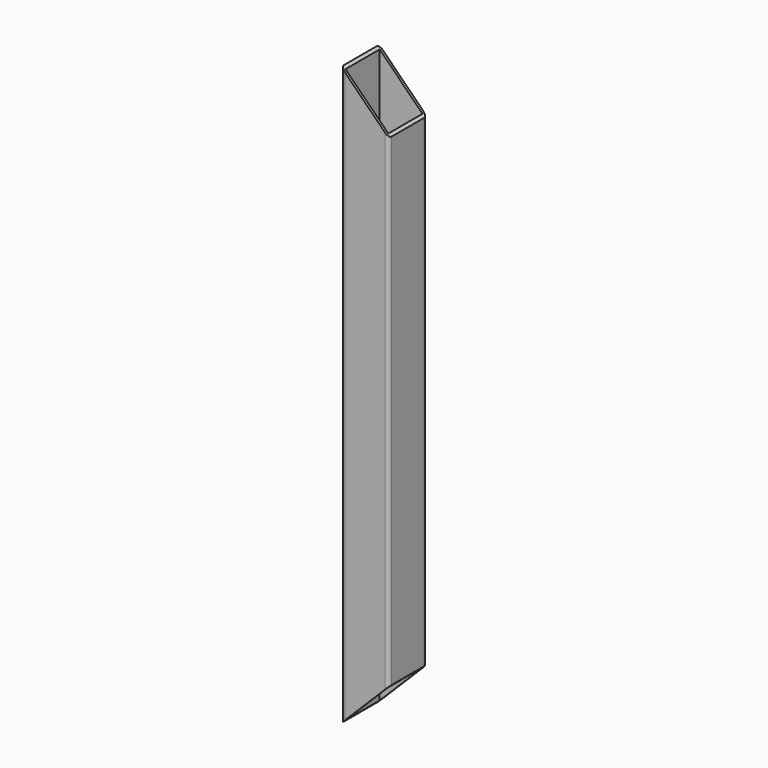
from build123d import *

# Parameters (mm, degrees)
F0_W     = 36
F0_H     = 36
F1_DEPTH = 243
F3_DEPTH = 40.001


# Not quite as in the source:
# - a pattern or mirror of a feature is missing from the dataset's text; its kind, count and spacing are read off the source's solid


with BuildPart() as f1:
    # F0 (on Top) → F1 (new body, symmetric)
    with BuildSketch(Plane.XY):
        with BuildLine():
            Line((17, 20), (-17, 20))
            ThreePointArc((-17, 20), (-19.1213203436, 19.1213203436), (-20, 17))
            Line((-20, 17), (-20, -17))
            ThreePointArc((-20, -17), (-19.1213203436, -19.1213203436), (-17, -20))
            Line((-17, -20), (17, -20))
            ThreePointArc((17, -20), (19.1213203436, -19.1213203436), (20, -17))
            Line((20, -17), (20, 17))
            ThreePointArc((20, 17), (19.1213203436, 19.1213203436), (17, 20))
        make_face()
        Rectangle(F0_W, F0_H, mode=Mode.SUBTRACT)
    extrude(amount=F1_DEPTH, both=True)

    # F2 (on face) → F3 (cut, through all)
    with BuildSketch(Plane.XZ.offset(20)):
        Polygon((20, 243), (-20, 243), (20, 203), align=None)
    f3 = extrude(amount=-F3_DEPTH, mode=Mode.SUBTRACT)

    # F3_copies: F3 across plane
    add(f3.mirror(Plane(origin=(0, 0, 0), x_dir=(-1, 0, 0), z_dir=(0, 0, -1))), mode=Mode.SUBTRACT)


solid = f1.part
